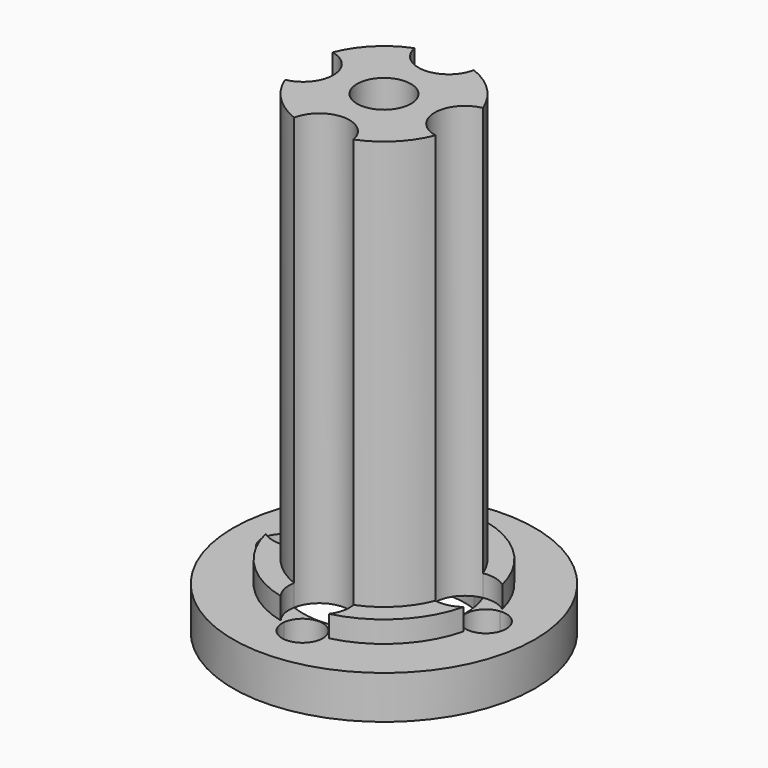
from build123d import *

# Parameters (mm, degrees)
F0_R     = 8.89
F1_DEPTH = 2.54
F0_R_2   = 1.5875
F2_DEPTH = 25.4
F3_DEPTH = 1.27


# Not quite as in the source:
# - a feature names something its author has since deleted; it is built from what else it names


with BuildPart() as f1:
    # F0 (on Top) → F1 (new body)
    with BuildSketch(Plane.XY):
        Circle(F0_R)
        with BuildLine():
            ThreePointArc((1.4227110748, 5.8288851076), (4.2426411821, 4.2426411821), (5.8288851076, 1.4227110748))
            ThreePointArc((5.8288851076, 1.4227110748), (5.8555597964, 1.3085976735), (5.880000686, 1.1939850638))
            ThreePointArc((5.880000686, 1.1939850638), (6.8049852658, 0.8899439223), (7.20000084, 0))
            ThreePointArc((7.20000084, 0), (6.8049852658, -0.8899439223), (5.880000686, -1.1939850638))
            ThreePointArc((5.880000686, -1.1939850638), (5.8555597964, -1.3085976735), (5.8288851076, -1.4227110748))
            ThreePointArc((5.8288851076, -1.4227110748), (4.2426411821, -4.2426411821), (1.4227110748, -5.8288851076))
            ThreePointArc((1.4227110748, -5.8288851076), (1.3085976735, -5.8555597964), (1.1939850638, -5.880000686))
            ThreePointArc((1.1939850638, -5.880000686), (1.1984954276, -5.9399253629), (1.20000014, -6.0000007))
            ThreePointArc((1.20000014, -6.0000007), (-0.0600753371, -7.1984961276), (-1.1939850638, -5.880000686))
            ThreePointArc((-1.1939850638, -5.880000686), (-1.3085976735, -5.8555597964), (-1.4227110748, -5.8288851076))
            ThreePointArc((-1.4227110748, -5.8288851076), (-4.2426411821, -4.2426411821), (-5.8288851076, -1.4227110748))
            ThreePointArc((-5.8288851076, -1.4227110748), (-5.8555597964, -1.3085976735), (-5.880000686, -1.1939850638))
            ThreePointArc((-5.880000686, -1.1939850638), (-7.20000084, 0), (-5.880000686, 1.1939850638))
            ThreePointArc((-5.880000686, 1.1939850638), (-5.8555597964, 1.3085976735), (-5.8288851076, 1.4227110748))
            ThreePointArc((-5.8288851076, 1.4227110748), (-4.2426411821, 4.2426411821), (-1.4227110748, 5.8288851076))
            ThreePointArc((-1.4227110748, 5.8288851076), (-1.3085976735, 5.8555597964), (-1.1939850638, 5.880000686))
            ThreePointArc((-1.1939850638, 5.880000686), (-0.0600753371, 7.1984961276), (1.20000014, 6.0000007))
            ThreePointArc((1.20000014, 6.0000007), (1.1984954276, 5.9399253629), (1.1939850638, 5.880000686))
            ThreePointArc((1.1939850638, 5.880000686), (1.3085976735, 5.8555597964), (1.4227110748, 5.8288851076))
        make_face(mode=Mode.SUBTRACT)
        with BuildLine():
            ThreePointArc((-4.4306066667, 1.7467486411), (-3.3675960454, 3.3675960454), (-1.7467486411, 4.4306066667))
            ThreePointArc((-1.7467486411, 4.4306066667), (-1.7320982571, 5.1638970948), (-1.4227110748, 5.8288851076))
            ThreePointArc((-1.4227110748, 5.8288851076), (-4.2426411821, 4.2426411821), (-5.8288851076, 1.4227110748))
            ThreePointArc((-5.8288851076, 1.4227110748), (-5.1638970948, 1.7320982571), (-4.4306066667, 1.7467486411))
        make_face()
        with BuildLine():
            ThreePointArc((1.7467486411, 4.4306066667), (3.3675960454, 3.3675960454), (4.4306066667, 1.7467486411))
            ThreePointArc((4.4306066667, 1.7467486411), (5.1638970948, 1.7320982571), (5.8288851076, 1.4227110748))
            ThreePointArc((5.8288851076, 1.4227110748), (4.2426411821, 4.2426411821), (1.4227110748, 5.8288851076))
            ThreePointArc((1.4227110748, 5.8288851076), (1.7320982571, 5.1638970948), (1.7467486411, 4.4306066667))
        make_face()
        with BuildLine():
            ThreePointArc((5.8288851076, -1.4227110748), (5.1638970948, -1.7320982571), (4.4306066667, -1.7467486411))
            ThreePointArc((4.4306066667, -1.7467486411), (3.3675960454, -3.3675960454), (1.7467486411, -4.4306066667))
            ThreePointArc((1.7467486411, -4.4306066667), (1.7320982571, -5.1638970948), (1.4227110748, -5.8288851076))
            ThreePointArc((1.4227110748, -5.8288851076), (4.2426411821, -4.2426411821), (5.8288851076, -1.4227110748))
        make_face()
        with BuildLine():
            ThreePointArc((-1.4227110748, -5.8288851076), (-1.7320982571, -5.1638970948), (-1.7467486411, -4.4306066667))
            ThreePointArc((-1.7467486411, -4.4306066667), (-3.3675960454, -3.3675960454), (-4.4306066667, -1.7467486411))
            ThreePointArc((-4.4306066667, -1.7467486411), (-5.1638970948, -1.7320982571), (-5.8288851076, -1.4227110748))
            ThreePointArc((-5.8288851076, -1.4227110748), (-4.2426411821, -4.2426411821), (-1.4227110748, -5.8288851076))
        make_face()
        with BuildLine():
            ThreePointArc((-1.7467486411, 4.4306066667), (0, 4.7625), (1.7467486411, 4.4306066667))
            ThreePointArc((1.7467486411, 4.4306066667), (1.7320982571, 5.1638970948), (1.4227110748, 5.8288851076))
            ThreePointArc((1.4227110748, 5.8288851076), (1.3085976735, 5.8555597964), (1.1939850638, 5.880000686))
            ThreePointArc((1.1939850638, 5.880000686), (0, 4.80000056), (-1.1939850638, 5.880000686))
            ThreePointArc((-1.1939850638, 5.880000686), (-1.3085976735, 5.8555597964), (-1.4227110748, 5.8288851076))
            ThreePointArc((-1.4227110748, 5.8288851076), (-1.7320982571, 5.1638970948), (-1.7467486411, 4.4306066667))
        make_face()
        with BuildLine():
            ThreePointArc((4.4306066667, 1.7467486411), (4.678791003, 0.889), (4.7625, 0))
            ThreePointArc((4.7625, 0), (4.678791003, -0.889), (4.4306066667, -1.7467486411))
            ThreePointArc((4.4306066667, -1.7467486411), (5.1638970948, -1.7320982571), (5.8288851076, -1.4227110748))
            ThreePointArc((5.8288851076, -1.4227110748), (5.8555597964, -1.3085976735), (5.880000686, -1.1939850638))
            ThreePointArc((5.880000686, -1.1939850638), (4.80000056, 0), (5.880000686, 1.1939850638))
            ThreePointArc((5.880000686, 1.1939850638), (5.8555597964, 1.3085976735), (5.8288851076, 1.4227110748))
            ThreePointArc((5.8288851076, 1.4227110748), (5.1638970948, 1.7320982571), (4.4306066667, 1.7467486411))
        make_face()
        with BuildLine():
            ThreePointArc((1.4227110748, -5.8288851076), (1.7320982571, -5.1638970948), (1.7467486411, -4.4306066667))
            ThreePointArc((1.7467486411, -4.4306066667), (0, -4.7625), (-1.7467486411, -4.4306066667))
            ThreePointArc((-1.7467486411, -4.4306066667), (-1.7320982571, -5.1638970948), (-1.4227110748, -5.8288851076))
            ThreePointArc((-1.4227110748, -5.8288851076), (-1.3085976735, -5.8555597964), (-1.1939850638, -5.880000686))
            ThreePointArc((-1.1939850638, -5.880000686), (0, -4.80000056), (1.1939850638, -5.880000686))
            ThreePointArc((1.1939850638, -5.880000686), (1.3085976735, -5.8555597964), (1.4227110748, -5.8288851076))
        make_face()
        with BuildLine():
            ThreePointArc((-4.4306066667, -1.7467486411), (-4.7625, 0), (-4.4306066667, 1.7467486411))
            ThreePointArc((-4.4306066667, 1.7467486411), (-5.1638970948, 1.7320982571), (-5.8288851076, 1.4227110748))
            ThreePointArc((-5.8288851076, 1.4227110748), (-5.8555597964, 1.3085976735), (-5.880000686, 1.1939850638))
            ThreePointArc((-5.880000686, 1.1939850638), (-5.1100567777, 0.8049845658), (-4.80000056, 0))
            ThreePointArc((-4.80000056, 0), (-5.1100567777, -0.8049845658), (-5.880000686, -1.1939850638))
            ThreePointArc((-5.880000686, -1.1939850638), (-5.8555597964, -1.3085976735), (-5.8288851076, -1.4227110748))
            ThreePointArc((-5.8288851076, -1.4227110748), (-5.1638970948, -1.7320982571), (-4.4306066667, -1.7467486411))
        make_face()
    extrude(amount=-F1_DEPTH)


with BuildPart() as f2:
    # F0 (on Top) → F2 (new body)
    with BuildSketch(Plane.XY):
        with BuildLine():
            ThreePointArc((4.4306066667, -1.7467486411), (2.9845, 0), (4.4306066667, 1.7467486411))
            ThreePointArc((4.4306066667, 1.7467486411), (3.3675960454, 3.3675960454), (1.7467486411, 4.4306066667))
            ThreePointArc((1.7467486411, 4.4306066667), (0, 2.9845), (-1.7467486411, 4.4306066667))
            ThreePointArc((-1.7467486411, 4.4306066667), (-3.3675960454, 3.3675960454), (-4.4306066667, 1.7467486411))
            ThreePointArc((-4.4306066667, 1.7467486411), (-2.9845, 0), (-4.4306066667, -1.7467486411))
            ThreePointArc((-4.4306066667, -1.7467486411), (-3.3675960454, -3.3675960454), (-1.7467486411, -4.4306066667))
            ThreePointArc((-1.7467486411, -4.4306066667), (0, -2.9845), (1.7467486411, -4.4306066667))
            ThreePointArc((1.7467486411, -4.4306066667), (3.3675960454, -3.3675960454), (4.4306066667, -1.7467486411))
        make_face()
        Circle(F0_R_2, mode=Mode.SUBTRACT)
    extrude(amount=F2_DEPTH)


with BuildPart() as f3:
    # F0 (on Top) → F3 (new body)
    with BuildSketch(Plane.XY):
        with BuildLine():
            ThreePointArc((-1.4227110748, -5.8288851076), (-1.7320982571, -5.1638970948), (-1.7467486411, -4.4306066667))
            ThreePointArc((-1.7467486411, -4.4306066667), (-3.3675960454, -3.3675960454), (-4.4306066667, -1.7467486411))
            ThreePointArc((-4.4306066667, -1.7467486411), (-5.1638970948, -1.7320982571), (-5.8288851076, -1.4227110748))
            ThreePointArc((-5.8288851076, -1.4227110748), (-4.2426411821, -4.2426411821), (-1.4227110748, -5.8288851076))
        make_face()
    extrude(amount=F3_DEPTH)


with BuildPart() as f3b:
    # F0 (on Top) → F3, piece 2 (new body)
    with BuildSketch(Plane.XY):
        with BuildLine():
            ThreePointArc((5.8288851076, -1.4227110748), (5.1638970948, -1.7320982571), (4.4306066667, -1.7467486411))
            ThreePointArc((4.4306066667, -1.7467486411), (3.3675960454, -3.3675960454), (1.7467486411, -4.4306066667))
            ThreePointArc((1.7467486411, -4.4306066667), (1.7320982571, -5.1638970948), (1.4227110748, -5.8288851076))
            ThreePointArc((1.4227110748, -5.8288851076), (4.2426411821, -4.2426411821), (5.8288851076, -1.4227110748))
        make_face()
    extrude(amount=F3_DEPTH)


with BuildPart() as f3c:
    # F0 (on Top) → F3, piece 3 (new body)
    with BuildSketch(Plane.XY):
        with BuildLine():
            ThreePointArc((1.7467486411, 4.4306066667), (3.3675960454, 3.3675960454), (4.4306066667, 1.7467486411))
            ThreePointArc((4.4306066667, 1.7467486411), (5.1638970948, 1.7320982571), (5.8288851076, 1.4227110748))
            ThreePointArc((5.8288851076, 1.4227110748), (4.2426411821, 4.2426411821), (1.4227110748, 5.8288851076))
            ThreePointArc((1.4227110748, 5.8288851076), (1.7320982571, 5.1638970948), (1.7467486411, 4.4306066667))
        make_face()
    extrude(amount=F3_DEPTH)


with BuildPart() as f3d:
    # F0 (on Top) → F3, piece 4 (new body)
    with BuildSketch(Plane.XY):
        with BuildLine():
            ThreePointArc((-4.4306066667, 1.7467486411), (-3.3675960454, 3.3675960454), (-1.7467486411, 4.4306066667))
            ThreePointArc((-1.7467486411, 4.4306066667), (-1.7320982571, 5.1638970948), (-1.4227110748, 5.8288851076))
            ThreePointArc((-1.4227110748, 5.8288851076), (-4.2426411821, 4.2426411821), (-5.8288851076, 1.4227110748))
            ThreePointArc((-5.8288851076, 1.4227110748), (-5.1638970948, 1.7320982571), (-4.4306066667, 1.7467486411))
        make_face()
    extrude(amount=F3_DEPTH)


solid = Compound([f1.part, f2.part, f3.part, f3b.part, f3c.part, f3d.part])
